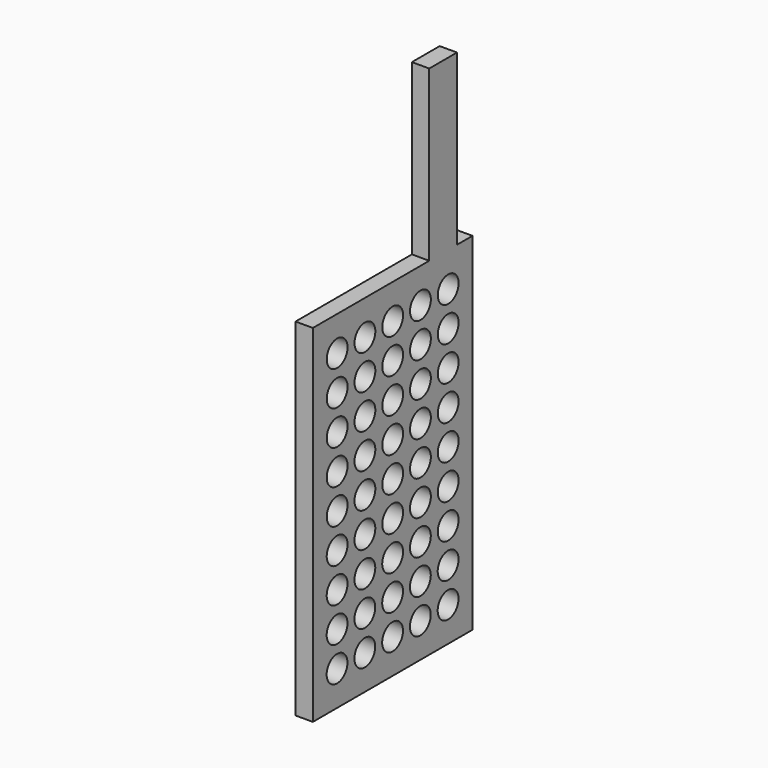
from build123d import *

# Parameters (mm, degrees)
F0_R     = 0.75
F0_W     = 2
F0_H     = 9.755
F1_DEPTH = 1


# Not quite as in the source:
# - a feature names something its author has since deleted; it is built from what else it names


with BuildPart() as f1:
    # F0 (on Right) → F1 (new body)
    with BuildSketch(Plane.YZ):
        Polygon((0, 0.245), (0, 0), (0, -19.7439561955), (11.5, -19.7439561955), (11.5, 0), (11.5, 0.245), (10.384144865, 0.245), (8.384144865, 0.245), (1.75, 0.245), align=None)
        with Locations((1.7424730282, -17.7489561955)):
            Circle(F0_R, mode=Mode.SUBTRACT)
        with Locations((1.7446237513, -15.7489573519)):
            Circle(F0_R, mode=Mode.SUBTRACT)
        with Locations((1.7467744744, -13.7489585083)):
            Circle(F0_R, mode=Mode.SUBTRACT)
        with Locations((3.7424718718, -17.7511069186)):
            Circle(F0_R, mode=Mode.SUBTRACT)
        with Locations((5.7424707154, -17.7532576417)):
            Circle(F0_R, mode=Mode.SUBTRACT)
        with Locations((3.7446225949, -15.751108075)):
            Circle(F0_R, mode=Mode.SUBTRACT)
        with Locations((3.746773318, -13.7511092314)):
            Circle(F0_R, mode=Mode.SUBTRACT)
        with Locations((5.7446214385, -15.7532587981)):
            Circle(F0_R, mode=Mode.SUBTRACT)
        with Locations((5.7467721616, -13.7532599545)):
            Circle(F0_R, mode=Mode.SUBTRACT)
        with Locations((1.7489251975, -11.7489596647)):
            Circle(F0_R, mode=Mode.SUBTRACT)
        with Locations((1.75, -9.75)):
            Circle(F0_R, mode=Mode.SUBTRACT)
        with Locations((1.75, -7.75)):
            Circle(F0_R, mode=Mode.SUBTRACT)
        with Locations((1.75, -5.75)):
            Circle(F0_R, mode=Mode.SUBTRACT)
        with Locations((3.7489243397, -11.7505550493)):
            Circle(F0_R, mode=Mode.SUBTRACT)
        with Locations((3.7499997014, -9.7505553384)):
            Circle(F0_R, mode=Mode.SUBTRACT)
        with Locations((5.7489228847, -11.7532611109)):
            Circle(F0_R, mode=Mode.SUBTRACT)
        with Locations((3.75, -7.75)):
            Circle(F0_R, mode=Mode.SUBTRACT)
        with Locations((3.75, -5.75)):
            Circle(F0_R, mode=Mode.SUBTRACT)
        with Locations((7.742469559, -17.7554083647)):
            Circle(F0_R, mode=Mode.SUBTRACT)
        with Locations((7.7446202821, -15.7554095212)):
            Circle(F0_R, mode=Mode.SUBTRACT)
        with Locations((7.7467710052, -13.7554106776)):
            Circle(F0_R, mode=Mode.SUBTRACT)
        with Locations((9.7424684026, -17.7575590878)):
            Circle(F0_R, mode=Mode.SUBTRACT)
        with Locations((9.7446191257, -15.7575602442)):
            Circle(F0_R, mode=Mode.SUBTRACT)
        with Locations((9.7467698488, -13.7575614006)):
            Circle(F0_R, mode=Mode.SUBTRACT)
        with Locations((5.75, -9.75)):
            Circle(F0_R, mode=Mode.SUBTRACT)
        with Locations((7.7489217283, -11.755411834)):
            Circle(F0_R, mode=Mode.SUBTRACT)
        with Locations((7.75, -9.75)):
            Circle(F0_R, mode=Mode.SUBTRACT)
        with Locations((5.75, -7.75)):
            Circle(F0_R, mode=Mode.SUBTRACT)
        with Locations((5.75, -5.75)):
            Circle(F0_R, mode=Mode.SUBTRACT)
        with Locations((7.75, -7.75)):
            Circle(F0_R, mode=Mode.SUBTRACT)
        with Locations((7.75, -5.75)):
            Circle(F0_R, mode=Mode.SUBTRACT)
        with Locations((9.7489205719, -11.7575625571)):
            Circle(F0_R, mode=Mode.SUBTRACT)
        with Locations((9.75, -9.75)):
            Circle(F0_R, mode=Mode.SUBTRACT)
        with Locations((9.75, -7.75)):
            Circle(F0_R, mode=Mode.SUBTRACT)
        with Locations((9.75, -5.75)):
            Circle(F0_R, mode=Mode.SUBTRACT)
        with Locations((1.75, -3.75)):
            Circle(F0_R, mode=Mode.SUBTRACT)
        with Locations((1.75, -1.75)):
            Circle(F0_R, mode=Mode.SUBTRACT)
        with Locations((3.75, -3.75)):
            Circle(F0_R, mode=Mode.SUBTRACT)
        with Locations((3.75, -1.75)):
            Circle(F0_R, mode=Mode.SUBTRACT)
        with Locations((5.75, -3.75)):
            Circle(F0_R, mode=Mode.SUBTRACT)
        with Locations((5.75, -1.75)):
            Circle(F0_R, mode=Mode.SUBTRACT)
        with Locations((7.75, -3.75)):
            Circle(F0_R, mode=Mode.SUBTRACT)
        with Locations((7.7499570354, -1.7564534015)):
            Circle(F0_R, mode=Mode.SUBTRACT)
        with Locations((9.75, -3.75)):
            Circle(F0_R, mode=Mode.SUBTRACT)
        with Locations((9.75, -1.75)):
            Circle(F0_R, mode=Mode.SUBTRACT)
        with Locations((9.384144865, 5.1225)):
            Rectangle(F0_W, F0_H)
    extrude(amount=F1_DEPTH)


solid = f1.part
